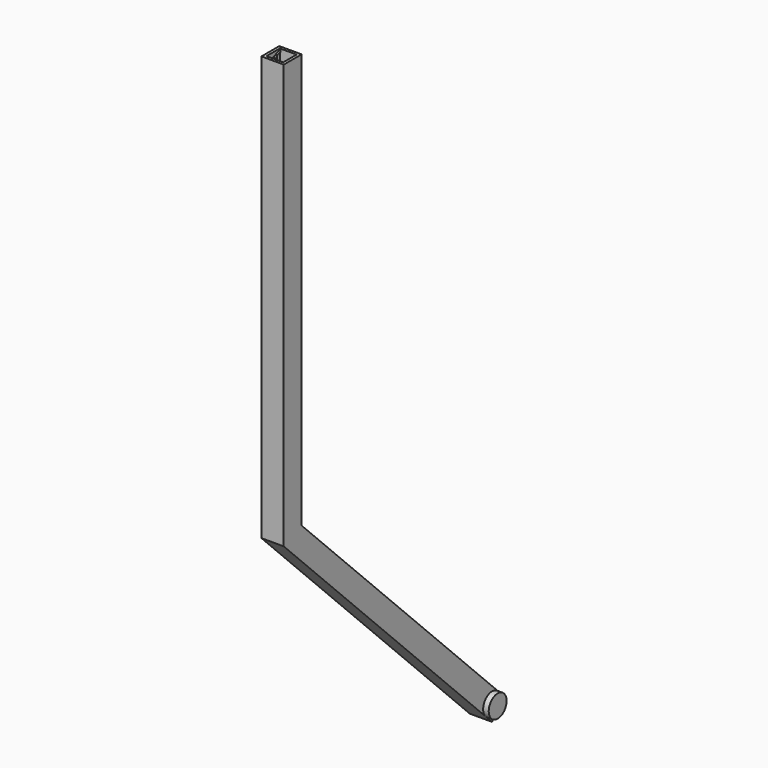
from build123d import *

# Parameters (mm, degrees)
F1_DEPTH     = 20
F3_DEPTH     = 5
F5_W         = 15
F5_H         = 15
F6_DEPTH     = 100
F7_TEXT_SIZE = 25.7612516483
F8_DEPTH     = 3


# Not quite as in the source:
# - Text() gives the source's letters only with a copy of the font that has no kerning and outlines rounded to 1/6400 em; it was checked with that copy


with BuildPart() as f1:
    # F0 (on Right) → F1 (new body)
    with BuildSketch(Plane.YZ):
        Polygon((-53.8653362151, 203.3568546289), (-73.8653362151, 203.3568546289), (-73.8653362151, -176.6431453711), (-53.8653362151, -168.3588741236), align=None)
        Polygon((-53.8653362151, -168.3588741236), (-73.8653362151, -176.6431453711), (159.4799015765, -409.9883831626), (173.6220372002, -395.8462475389), align=None)
    extrude(amount=F1_DEPTH)

    # F2 (on face) → F3 (join)
    with BuildSketch(Plane.YZ.offset(20)):
        with BuildLine():
            ThreePointArc((166.55096926, -402.9173154791), (168.7186968668, -399.6730819464), (169.4799015765, -395.8462475389))
            ThreePointArc((169.4799015765, -395.8462475389), (168.7186969016, -392.0194132152), (166.5509693883, -388.775179727))
            ThreePointArc((166.5509693883, -388.775179727), (152.408833765, -388.7751797267), (152.4088337639, -402.91731535))
            ThreePointArc((152.4088337639, -402.91731535), (159.4799014852, -405.8462475389), (166.55096926, -402.9173154791))
        make_face()
    extrude(amount=F3_DEPTH)

    # F5 (on face) → F6 (cut)
    with BuildSketch(Plane.XY.offset(203.3568546289)):
        with Locations((10, -63.8653362151)):
            Rectangle(F5_W, F5_H)
    extrude(amount=-F6_DEPTH, mode=Mode.SUBTRACT)

    # F7 (on face) → F8 (cut)
    with BuildSketch(Plane(origin=(0, 0, 0), x_dir=(0, -1, 0), z_dir=(-1, 0, 0))):
        with Locations(Location((53.8653362151, 203.3568546289), (0, 0, -90))):
            Text('ALTO 2', F7_TEXT_SIZE, font='Open Sans', text_align=(TextAlign.LEFT, TextAlign.BOTTOM))
    extrude(amount=-F8_DEPTH, mode=Mode.SUBTRACT)


solid = f1.part
